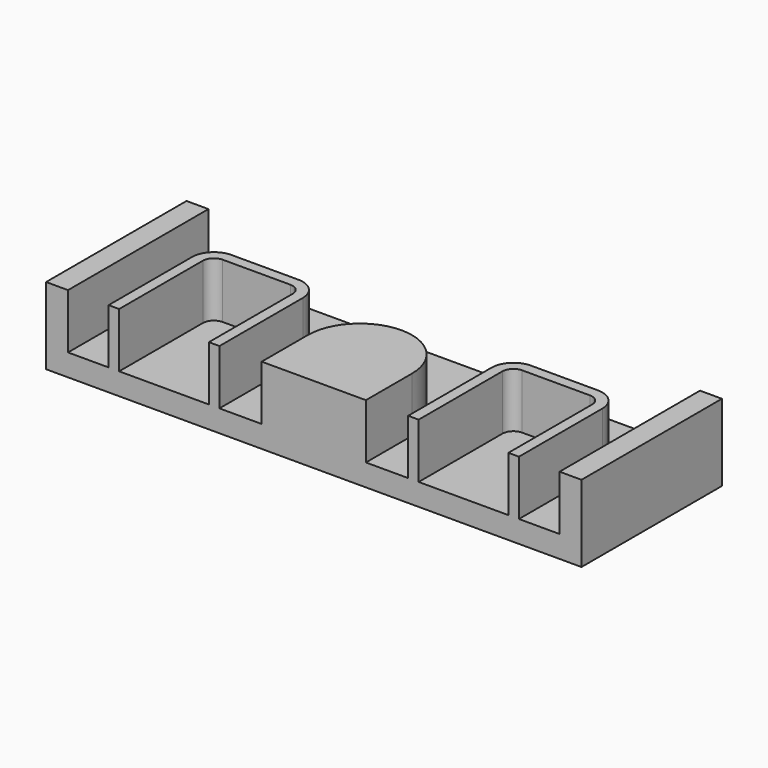
from build123d import *

# Parameters (mm, degrees)
F0_W     = 44.8
F0_H     = 16
F1_DEPTH = 2
F4_DEPTH = 5
F5_DEPTH = 5
F6_W     = 2
F6_H     = 16
F7_DEPTH = 7


# Not quite as in the source:
# - a pattern or mirror of a feature is missing from the dataset's text; its kind, count and spacing are read off the source's solid


with BuildPart() as f1:
    # F0 (on Top) → F1 (new body)
    with BuildSketch(Plane.XY):
        Rectangle(F0_W, F0_H)
    extrude(amount=F1_DEPTH)

    # F2 (on face) → F4 (join)
    with BuildSketch(Plane.XY.offset(2)):
        with BuildLine():
            Line((-18.7, 1.5), (-18.7, -8))
            Line((-18.7, -8), (-17.74, -8))
            Line((-17.74, -8), (-17.74, 1.54))
            ThreePointArc((-17.74, 1.54), (-17.4471067812, 2.2471067812), (-16.74, 2.54))
            Line((-16.74, 2.54), (-10.56, 2.54))
            ThreePointArc((-10.56, 2.54), (-9.8528932188, 2.2471067812), (-9.56, 1.54))
            Line((-9.56, 1.54), (-9.56, -8))
            Line((-9.56, -8), (-8.6, -8))
            Line((-8.6, -8), (-8.6, 1.5))
            ThreePointArc((-8.6, 1.5), (-9.1857864376, 2.9142135624), (-10.6, 3.5))
            Line((-10.6, 3.5), (-16.7, 3.5))
            ThreePointArc((-16.7, 3.5), (-18.1142135624, 2.9142135624), (-18.7, 1.5))
        make_face()
    f4 = extrude(amount=F4_DEPTH)

    # F4_copies: F4 across plane
    add(f4.mirror(Plane(origin=(0, 0, 0), x_dir=(0, 0, 1), z_dir=(1, 0, 0))))

    # F3 (on face) → F5 (join)
    with BuildSketch(Plane.XY.offset(2)):
        with BuildLine():
            Line((4.75, -8), (4.75, -2.75))
            ThreePointArc((4.75, -2.75), (0, 2), (-4.75, -2.75))
            Line((-4.75, -2.75), (-4.75, -8))
            Line((-4.75, -8), (4.75, -8))
        make_face()
    extrude(amount=F5_DEPTH)

    # F6 (on Top) → F7 (join, through all)
    with BuildSketch(Plane.XY):
        with Locations((-23.4, 0)):
            Rectangle(F6_W, F6_H)
    f7 = extrude(amount=F7_DEPTH)

    # F7_copies: F7 across plane
    add(f7.mirror(Plane(origin=(0, 0, 0), x_dir=(0, 0, 1), z_dir=(1, 0, 0))))


solid = f1.part
